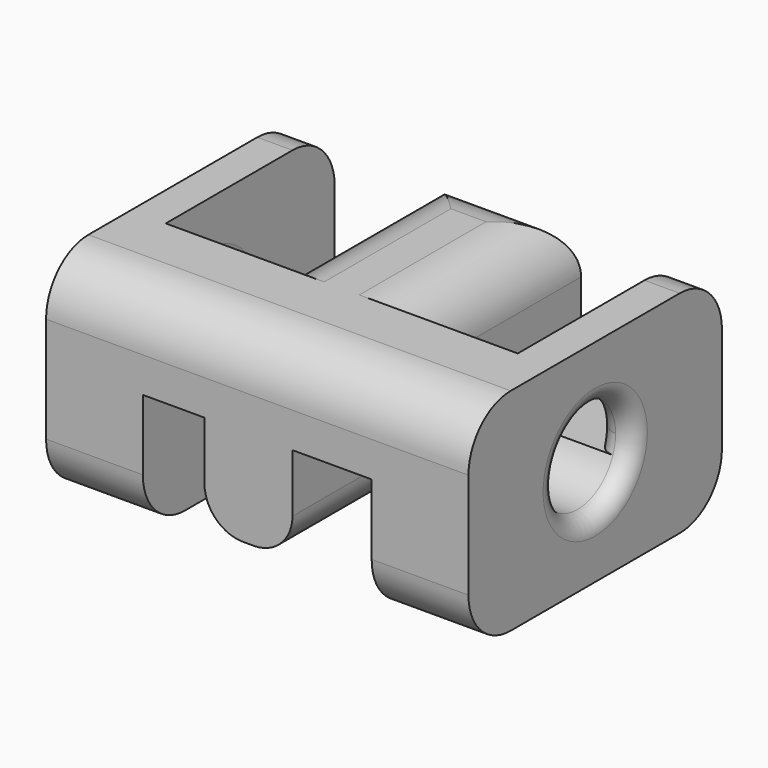
from build123d import *

# Parameters (mm, degrees)
F0_W          = 12
F0_H          = 9
F1_DEPTH      = 6
F2_W          = 3
F2_H          = 6
F3_DEPTH      = 3.5
F4_W          = 6.5
F4_H          = 6.5
F5_DEPTH      = 3.5
F6_R          = 1.35
F7_DEPTH      = 3
F8_R          = 1.25
F9_DEPTH      = 2.751
F10_R         = 1.5
F11_W         = 2.5
F11_H         = 6.5
F12_DEPTH     = 2.75
F13_R         = 1.1
F14_T8_ANGLE  = 247.5355258221
F14_T13_ANGLE = 74.7913514773
F14_T18_ANGLE = 254.8973081934
F14_T24_ANGLE = 80.8755372564
F14_T30_ANGLE = 260.9918579461


# Not quite as in the source:
# - a fillet or chamfer that OpenCascade refuses, or shapes differently, is made with other operations: its cross-section is extruded or revolved along the edge and cut away or added


with BuildPart() as f1:
    # F0 (on Top) → F1 (new body)
    with BuildSketch(Plane.XY):
        Rectangle(F0_W, F0_H)
    extrude(amount=F1_DEPTH)

    # F2 (on face) → F3 (cut)
    with BuildSketch(Plane.XY.offset(6)):
        with Locations((3.5, 1.5)):
            Rectangle(F2_W, F2_H)
        with Locations((-3.5, 1.5)):
            Rectangle(F2_W, F2_H)
    extrude(amount=-F3_DEPTH, mode=Mode.SUBTRACT)

    # F4 (on face) → F5 (cut)
    with BuildSketch(Plane(origin=(0, 0, 0), x_dir=(1, 0, 0), z_dir=(0, 0, -1))):
        with Locations((0, 1.25)):
            Rectangle(F4_W, F4_H)
    extrude(amount=-F5_DEPTH, mode=Mode.SUBTRACT)

    # F6 (on face) → F7 (cut)
    with BuildSketch(Plane.YZ.offset(6)):
        with Locations((0, 3)):
            Circle(F6_R)
    extrude(amount=-F7_DEPTH, mode=Mode.SUBTRACT)

    # F8 (on face) → F9 (cut, through all)
    with BuildSketch(Plane(origin=(-6, 0, 0), x_dir=(0, -1, 0), z_dir=(-1, 0, 0))):
        with Locations((0, 3)):
            Circle(F8_R)
    extrude(amount=-F9_DEPTH, mode=Mode.SUBTRACT)

    # F10
    f10_edges = [f1.edges().sort_by_distance(p)[0] for p in [
        (2, 1.5, 6),
        (-2, 1.5, 6),
        (0, -4.5, 6),
        (-4.625, -4.5, 0),
        (4.625, -4.5, 0),
        (0, 4.5, 0),
        (-5.5, 4.5, 6),
        (5.5, 4.5, 6),
        (0, 4.5, 6),
    ]]
    fillet(f10_edges, radius=F10_R)

    # F11 (on face) → F12 (join)
    with BuildSketch(Plane(origin=(0, 0, 3.5), x_dir=(1, 0, 0), z_dir=(0, 0, -1))):
        with Locations((-0.25, 1.25)):
            Rectangle(F11_W, F11_H)
    extrude(amount=F12_DEPTH)

    # F13
    f13_edges = [f1.edges().sort_by_distance(p)[0] for p in [
        (-1.5, -1.25, 0.75),
        (1, -1.25, 0.75),
    ]]
    fillet(f13_edges, radius=F13_R)

    # F14: fillet of radius 0.5 on 7 edges, made by hand

    # F14_s1 → F14_t2 (revolve, cut)
    with BuildSketch(Plane.XY.offset(3)):
        with BuildLine():
            ThreePointArc((6, 1.85), (5.8535533906, 1.4964466094), (5.5, 1.35))
            Line((5.5, 1.35), (6, 1.35))
            Line((6, 1.35), (6, 1.85))
        make_face()
    revolve(axis=Axis((6, 0, 3), (1, 0, 0)), mode=Mode.SUBTRACT)

    # F14_s3 → F14_t4 (revolve, cut)
    with BuildSketch(Plane.XY.offset(3)):
        with BuildLine():
            ThreePointArc((-6, -1.75), (-5.8535533906, -1.3964466094), (-5.5, -1.25))
            Line((-5.5, -1.25), (-6, -1.25))
            Line((-6, -1.25), (-6, -1.75))
        make_face()
    revolve(axis=Axis((-6, 0, 3), (-1, 0, 0)), mode=Mode.SUBTRACT)


with BuildPart() as f14_tool6:
    # F14_s7 → F14_t8 (revolve)
    with BuildSketch(Plane(origin=(0, -1.3861749524, 2.0731657713), x_dir=(1, 0, 0), z_dir=(0, -0.5558279796, 0.8312973338))):
        with BuildLine():
            ThreePointArc((-3.25, 3.4174839388), (-3.3964466094, 3.0639305482), (-3.75, 2.9174839388))
            Line((-3.75, 2.9174839388), (-3.25, 2.9174839388))
            Line((-3.25, 2.9174839388), (-3.25, 3.4174839388))
        make_face()
    revolve(axis=Axis((-3.25, 0, 3), (-1, 0, 0)), revolution_arc=F14_T8_ANGLE)

    split(bisect_by=Plane.XY.offset(3.5), keep=Keep.BOTTOM)


with BuildPart() as f1_1:
    add(f1.part)

    # F14_t5: cut F14_tool6
    add(f14_tool6.part, mode=Mode.SUBTRACT)


with BuildPart() as f14_tool11:
    # F14_s12 → F14_t13 (revolve)
    with BuildSketch(Plane(origin=(0, 0.7594411885, 0.2064587052), x_dir=(1, 0, 0), z_dir=(0, -0.9649769073, -0.2623348403))):
        with BuildLine():
            ThreePointArc((5.5, 1.5449307218), (5.1464466094, 1.3984841124), (5, 1.0449307218))
            Line((5, 1.0449307218), (5, 1.5449307218))
            Line((5, 1.5449307218), (5.5, 1.5449307218))
        make_face()
    revolve(axis=Axis((5, 0, 3), (1, 0, 0)), revolution_arc=F14_T13_ANGLE)

    split(bisect_by=Plane.XY.offset(2.5), keep=Keep.TOP)


with BuildPart() as f1_2:
    add(f1_1.part)

    # F14_t10: cut F14_tool11
    add(f14_tool11.part, mode=Mode.SUBTRACT)


with BuildPart() as f14_tool16:
    # F14_s17 → F14_t18 (revolve)
    with BuildSketch(Plane.XY.offset(3)):
        with BuildLine():
            ThreePointArc((5.5, 1.35), (5.1464466094, 1.4964466094), (5, 1.85))
            Line((5, 1.85), (5, 1.35))
            Line((5, 1.35), (5.5, 1.35))
        make_face()
    revolve(axis=Axis((5, 0, 3), (1, 0, 0)), revolution_arc=F14_T18_ANGLE)

    split(bisect_by=Plane.XZ.offset(1.5), keep=Keep.BOTTOM)

    split(bisect_by=Plane.XY.offset(2.5), keep=Keep.TOP)


with BuildPart() as f1_3:
    add(f1_2.part)

    # F14_t15: cut F14_tool16
    add(f14_tool16.part, mode=Mode.SUBTRACT)


with BuildPart() as f14_tool22:
    # F14_s23 → F14_t24 (revolve)
    with BuildSketch(Plane(origin=(0, -0.469718994, 0.0754425014), x_dir=(1, 0, 0), z_dir=(0, 0.9873461903, -0.1585796345))):
        with BuildLine():
            ThreePointArc((-5.5, -1.7120385709), (-5.1464466094, -1.5655919615), (-5, -1.2120385709))
            Line((-5, -1.2120385709), (-5, -1.7120385709))
            Line((-5, -1.7120385709), (-5.5, -1.7120385709))
        make_face()
    revolve(axis=Axis((-5, 0, 3), (-1, 0, 0)), revolution_arc=F14_T24_ANGLE)

    split(bisect_by=Plane.XZ.offset(1.5), keep=Keep.BOTTOM)

    split(bisect_by=Plane.XY.offset(2.5), keep=Keep.TOP)


with BuildPart() as f1_4:
    add(f1_3.part)

    # F14_t21: cut F14_tool22
    add(f14_tool22.part, mode=Mode.SUBTRACT)


with BuildPart() as f14_tool28:
    # F14_s29 → F14_t30 (revolve)
    with BuildSketch(Plane.XY.offset(3)):
        with BuildLine():
            ThreePointArc((-5.5, -1.25), (-5.1464466094, -1.3964466094), (-5, -1.75))
            Line((-5, -1.75), (-5, -1.25))
            Line((-5, -1.25), (-5.5, -1.25))
        make_face()
    revolve(axis=Axis((-5, 0, 3), (-1, 0, 0)), revolution_arc=F14_T30_ANGLE)

    split(bisect_by=Plane.XZ.offset(1.5), keep=Keep.BOTTOM)

    split(bisect_by=Plane.XY.offset(2.5), keep=Keep.TOP)


with BuildPart() as f1_5:
    add(f1_4.part)

    # F14_t27: cut F14_tool28
    add(f14_tool28.part, mode=Mode.SUBTRACT)


solid = f1_5.part
